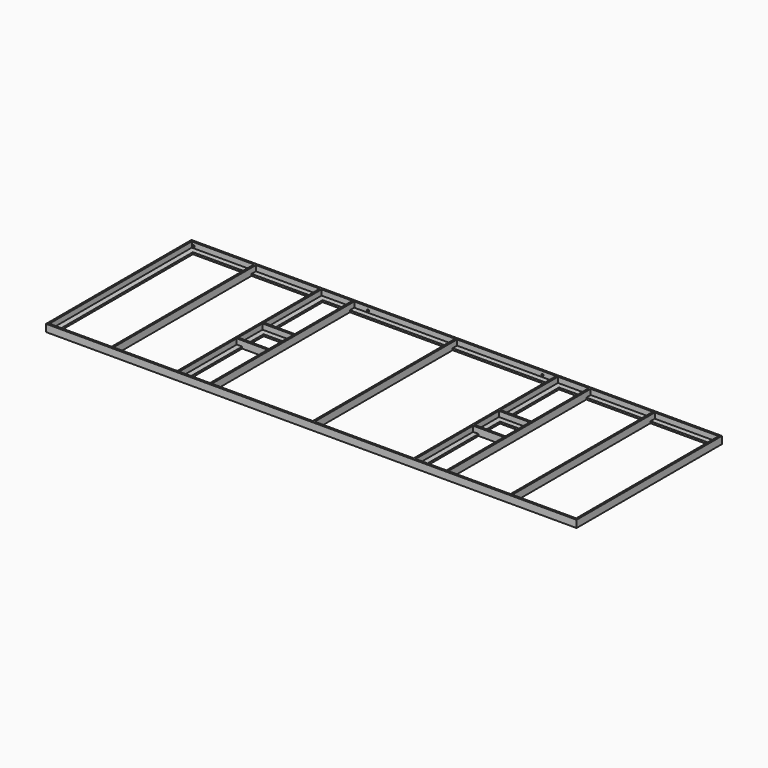
from build123d import *

# Parameters (mm, degrees)
F0_W      = 25.4
F0_H      = 25.4
F0_W_2    = 1803.4
F0_H_2    = 584.2
F1_DEPTH  = 25.4
F2_W      = 1841.5
F2_H      = 622.3
F2_W_2    = 1803.4
F2_H_2    = 584.2
F3_DEPTH  = 19.05
F4_W      = 25.4
F4_H      = 232.57764
F4_H_2    = 25.4
F4_W_2    = 69.8373
F4_H_3    = 68.24472
F5_DEPTH  = 25.4
F6_W      = 19.05
F6_H      = 251.62764
F6_W_2    = 107.9373
F6_H_2    = 106.34472
F6_W_3    = 69.8373
F6_H_3    = 68.24472
F7_DEPTH  = 19.05
F8_R      = 3.571875
F9_DEPTH  = 25.4
F10_R     = 3.5687
F11_DEPTH = 25.4
F12_W     = 6.35
F12_H     = 622.3
F13_DEPTH = 25.4


# Not quite as in the source:
# - a feature names something its author has since deleted; it is built from what else it names


with BuildPart() as f1:
    # F0 (on Top) → F1 (new body)
    with BuildSketch(Plane.XY):
        with Locations((12.7, -12.7)):
            Rectangle(F0_W, F0_H)
        with Locations((927.1, -12.7)):
            Rectangle(F0_W_2, F0_H)
        with Locations((12.7, -317.5)):
            Rectangle(F0_W, F0_H_2)
        with Locations((1841.5, -12.7)):
            Rectangle(F0_W, F0_H)
        with Locations((12.7, -622.3)):
            Rectangle(F0_W, F0_H)
        with Locations((1841.5, -317.5)):
            Rectangle(F0_W, F0_H_2)
        with Locations((927.1, -622.3)):
            Rectangle(F0_W_2, F0_H)
        with Locations((1841.5, -622.3)):
            Rectangle(F0_W, F0_H)
    extrude(amount=F1_DEPTH)

    # F2 (on face) → F3 (cut)
    with BuildSketch(Plane.XY.offset(25.4)):
        with Locations((927.1, -317.5)):
            Rectangle(F2_W, F2_H)
        with Locations((927.1, -317.5)):
            Rectangle(F2_W_2, F2_H_2, mode=Mode.SUBTRACT)
    extrude(amount=-F3_DEPTH, mode=Mode.SUBTRACT)

    # F4 (on face) → F5 (join)
    with BuildSketch(Plane(origin=(0, 0, 0), x_dir=(1, 0, 0), z_dir=(0, 0, -1))):
        with Locations((466.2932, 493.31118)):
            Rectangle(F4_W, F4_H)
        with Locations((466.2932, 622.3)):
            Rectangle(F4_W, F4_H_2)
        with Locations((561.5305, 622.3)):
            Rectangle(F4_W, F4_H_2)
        with Locations((561.5305, 493.31118)):
            Rectangle(F4_W, F4_H)
        with Locations((561.5305, 364.32236)):
            Rectangle(F4_W, F4_H_2)
        with Locations((513.91185, 364.32236)):
            Rectangle(F4_W_2, F4_H_2)
        with Locations((466.2932, 364.32236)):
            Rectangle(F4_W, F4_H_2)
        with Locations((466.2932, 317.5)):
            Rectangle(F4_W, F4_H_3)
        with Locations((561.5305, 317.5)):
            Rectangle(F4_W, F4_H_3)
        with Locations((561.5305, 270.67764)):
            Rectangle(F4_W, F4_H_2)
        with Locations((513.91185, 270.67764)):
            Rectangle(F4_W_2, F4_H_2)
        with Locations((466.2932, 270.67764)):
            Rectangle(F4_W, F4_H_2)
        with Locations((466.2932, 141.68882)):
            Rectangle(F4_W, F4_H)
        with Locations((466.2932, 12.7)):
            Rectangle(F4_W, F4_H_2)
        with Locations((561.5305, 12.7)):
            Rectangle(F4_W, F4_H_2)
        with Locations((561.5305, 141.68882)):
            Rectangle(F4_W, F4_H)
        with Locations((1292.6568, 317.5)):
            Rectangle(F4_W, F4_H_3)
        with Locations((1292.6568, 622.3)):
            Rectangle(F4_W, F4_H_2)
        with Locations((1387.8941, 622.3)):
            Rectangle(F4_W, F4_H_2)
        with Locations((1292.6568, 493.31118)):
            Rectangle(F4_W, F4_H)
        with Locations((1387.8941, 493.31118)):
            Rectangle(F4_W, F4_H)
        with Locations((1340.27545, 364.32236)):
            Rectangle(F4_W_2, F4_H_2)
        with Locations((1387.8941, 317.5)):
            Rectangle(F4_W, F4_H_3)
        with Locations((1387.8941, 364.32236)):
            Rectangle(F4_W, F4_H_2)
        with Locations((1292.6568, 364.32236)):
            Rectangle(F4_W, F4_H_2)
        with Locations((1292.6568, 270.67764)):
            Rectangle(F4_W, F4_H_2)
        with Locations((1340.27545, 270.67764)):
            Rectangle(F4_W_2, F4_H_2)
        with Locations((1387.8941, 270.67764)):
            Rectangle(F4_W, F4_H_2)
        with Locations((1387.8941, 141.68882)):
            Rectangle(F4_W, F4_H)
        with Locations((1292.6568, 141.68882)):
            Rectangle(F4_W, F4_H)
        with Locations((1292.6568, 12.7)):
            Rectangle(F4_W, F4_H_2)
        with Locations((1387.8941, 12.7)):
            Rectangle(F4_W, F4_H_2)
    extrude(amount=-F5_DEPTH)

    # F6 (on face) → F7 (cut)
    with BuildSketch(Plane.XY.offset(25.4)):
        with Locations((1295.8318, -132.16382)):
            Rectangle(F6_W, F6_H)
        with Locations((1384.7191, -132.16382)):
            Rectangle(F6_W, F6_H)
        with Locations((1340.27545, -317.5)):
            Rectangle(F6_W_2, F6_H_2)
        with Locations((1340.27545, -317.5)):
            Rectangle(F6_W_3, F6_H_3, mode=Mode.SUBTRACT)
        with Locations((1384.7191, -502.83618)):
            Rectangle(F6_W, F6_H)
        with Locations((1295.8318, -502.83618)):
            Rectangle(F6_W, F6_H)
        with Locations((558.3555, -502.83618)):
            Rectangle(F6_W, F6_H)
        with Locations((469.4682, -502.83618)):
            Rectangle(F6_W, F6_H)
        with Locations((513.91185, -317.5)):
            Rectangle(F6_W_2, F6_H_2)
        with Locations((513.91185, -317.5)):
            Rectangle(F6_W_3, F6_H_3, mode=Mode.SUBTRACT)
        with Locations((469.4682, -132.16382)):
            Rectangle(F6_W, F6_H)
        with Locations((558.3555, -132.16382)):
            Rectangle(F6_W, F6_H)
    extrude(amount=-F7_DEPTH, mode=Mode.SUBTRACT)

    # F8 (on face) → F9 (cut)
    with BuildSketch(Plane(origin=(0, 0, 0), x_dir=(1, 0, 0), z_dir=(0, 0, -1))):
        with Locations((12.7, 622.3)):
            Circle(F8_R)
        with Locations((622.3, 622.3)):
            Circle(F8_R)
        with Locations((1231.9, 622.3)):
            Circle(F8_R)
        with Locations((1841.5, 622.3)):
            Circle(F8_R)
    extrude(amount=-F9_DEPTH, mode=Mode.SUBTRACT)

    # F10 (on face) → F11 (cut)
    with BuildSketch(Plane(origin=(0, 0, 0), x_dir=(-1, 0, 0), z_dir=(0, 1, 0))):
        with Locations((-1841.5, 12.7)):
            Circle(F10_R)
        with Locations((-1231.9, 12.7)):
            Circle(F10_R)
        with Locations((-622.3, 12.7)):
            Circle(F10_R)
        with Locations((-12.7, 12.7)):
            Circle(F10_R)
    extrude(amount=-F11_DEPTH, mode=Mode.SUBTRACT)

    # F12 (on face) → F13 (join)
    with BuildSketch(Plane.XY.offset(25.4)):
        Polygon((230.3526, -6.35), (229.5906, -6.35), (224.0026, -6.35), (224.0026, -628.65), (229.5906, -628.65), (230.3526, -628.65), align=None)
        with Locations((930.26865, -317.5)):
            Rectangle(F12_W, F12_H)
        with Locations((1621.4471, -317.5)):
            Rectangle(F12_W, F12_H)
    extrude(amount=-F13_DEPTH)


solid = f1.part
